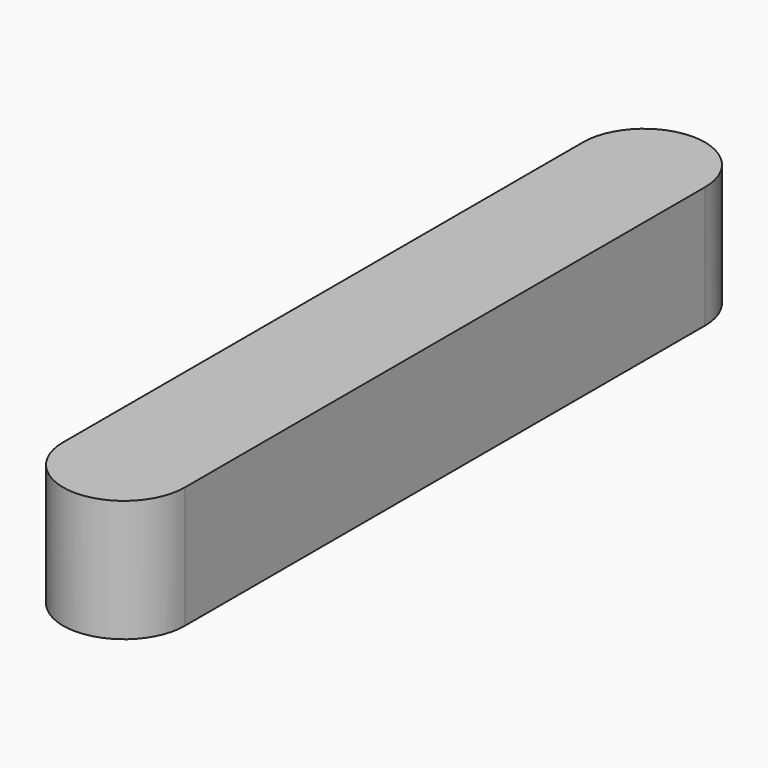
from build123d import *

# Parameters (mm, degrees)
F1_DEPTH = 9.525


# Not quite as in the source:
# - a length typed as a fraction of an inch, garbled in the dataset ("3 / 203.2 mm" for 3/8 in), is restored


with BuildPart() as f1:
    # F0 (on Top) → F1 (new body)
    with BuildSketch(Plane.XY):
        with BuildLine():
            ThreePointArc((-46.0191917587, 22.3519991428), (-50.7816917587, 27.1144991428), (-55.5441917587, 22.3519991428))
            Line((-55.5441917587, 22.3519991428), (-55.5441917587, -28.4480008572))
            ThreePointArc((-55.5441917587, -28.4480008572), (-50.7816917587, -33.2105008572), (-46.0191917587, -28.4480008572))
            Line((-46.0191917587, -28.4480008572), (-46.0191917587, 22.3519991428))
        make_face()
    extrude(amount=F1_DEPTH)


solid = f1.part
